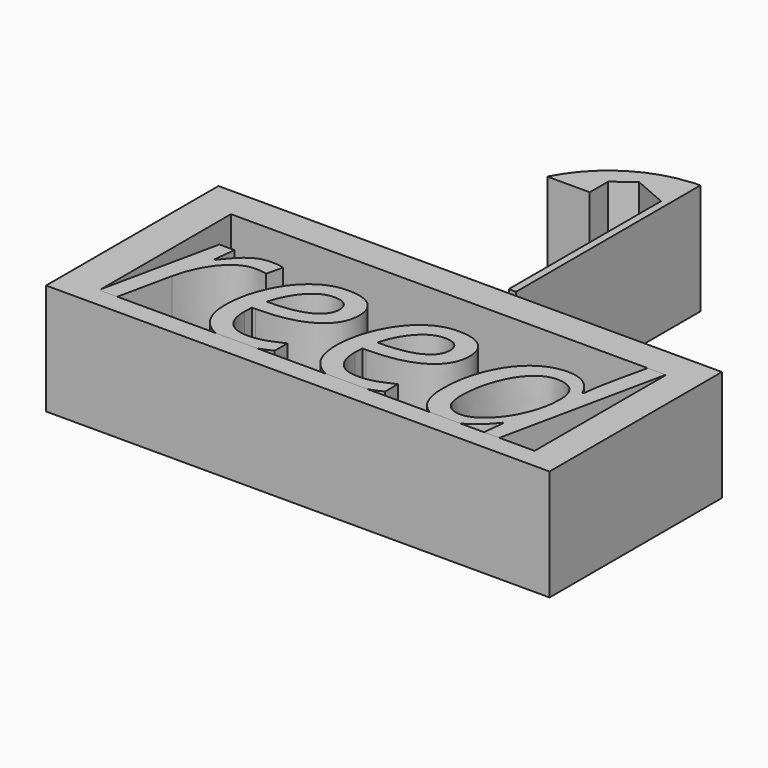
from build123d import *

# Parameters (mm, degrees)
F0_TEXT_SIZE = 51.2880169683
F1_DEPTH     = 25.4
F2_W         = 93.4035778046
F2_H         = 4.566386342
F2_W_2       = 6.2408708036
F2_W_3       = 99.6444486082
F2_H_2       = 7.1163624525
F2_W_4       = 1.6946494579
F2_W_5       = 7.0808120072
F3_DEPTH     = 25.4
F5_DEPTH     = 25.4


# Not quite as in the source:
# - Text() gives the source's letters only with a copy of the font that has no kerning and outlines rounded to 1/6400 em; it was checked with that copy


with BuildPart() as f1:
    # F0 (on Top) → F1 (new body)
    with BuildSketch(Plane.XY):
        with Locations((-53.9388656616, -75.9293287992)):
            Text('reed', F0_TEXT_SIZE, font='Open Sans', font_style=FontStyle.ITALIC, text_align=(TextAlign.LEFT, TextAlign.BOTTOM))
    extrude(amount=F1_DEPTH)


with BuildPart() as f3:
    # F2 (on Top) → F3 (new body)
    with BuildSketch(Plane.XY):
        with Locations((-5.6042224169, -77.9533907771)):
            Rectangle(F2_W, F2_H)
        Polygon((-52.3060113192, -80.2365839481), (-52.3060113192, -75.6701976061), (-52.3060113192, -38.0187183619), (-54.0006607771, -38.0187183619), (-54.0006607771, -80.2365839481), align=None)
        with Locations((44.2180018872, -77.9533907771)):
            Rectangle(F2_W_2, F2_H)
        with Locations((-2.4837870151, -34.4605371356)):
            Rectangle(F2_W_3, F2_H_2)
        with Locations((-53.1533360481, -34.4605371356)):
            Rectangle(F2_W_4, F2_H_2)
        Polygon((47.338437289, -38.0187183619), (47.338437289, -75.6701976061), (47.338437289, -80.2365839481), (54.4192492962, -80.2365839481), (54.4192492962, -38.0187183619), align=None)
        Polygon((-60.8616806567, -80.2365839481), (-54.0006607771, -80.2365839481), (-54.0006607771, -38.0187183619), (-54.0006607771, -30.9023559093), (-60.8616806567, -30.9023559093), align=None)
        with Locations((50.8788432926, -34.4605371356)):
            Rectangle(F2_W_5, F2_H_2)
    extrude(amount=F3_DEPTH)


with BuildPart() as f5:
    # F4 (on Top) → F5 (new body)
    with BuildSketch(Plane.XY):
        with BuildLine():
            Line((4.6046972275, -29.6465158463), (6.2791258097, -29.6465158463))
            Line((6.2791258097, -29.6465158463), (6.2791258097, 23.0982899666))
            ThreePointArc((6.2791258097, 23.0982899666), (5.441488901, 23.0849841514), (4.6046972275, 23.0450801326))
            Line((4.6046972275, 23.0450801326), (4.6046972275, 13.9426963335))
            Line((4.6046972275, 13.9426963335), (4.6046972275, -29.6465158463))
        make_face()
        with BuildLine():
            ThreePointArc((4.6046972275, 23.0450801326), (5.441488901, 23.0849841514), (6.2791258097, 23.0982899666))
            Line((6.2791258097, 23.0982899666), (4.6046972275, 23.0982899666))
            Line((4.6046972275, 23.0982899666), (4.6046972275, 23.0450801326))
        make_face()
        with BuildLine():
            Line((-3.0875055252, 17.2848684449), (4.6046972275, 13.9426963335))
            Line((4.6046972275, 13.9426963335), (4.6046972275, 23.0450801326))
            ThreePointArc((4.6046972275, 23.0450801326), (4.5661746808, 23.0426010171), (4.5276558042, 23.0400655174))
            Line((4.5276558042, 23.0400655174), (-3.0875055252, 17.2848684449))
        make_face()
        with BuildLine():
            Line((4.6046972275, 23.0450801326), (4.6046972275, 23.0982899666))
            Line((4.6046972275, 23.0982899666), (4.5276558042, 23.0400655174))
            ThreePointArc((4.5276558042, 23.0400655174), (4.5661746808, 23.0426010171), (4.6046972275, 23.0450801326))
        make_face()
        Polygon((-7.5098006262, 13.9426963335), (-3.0875055252, 17.2848684449), (-7.5098006262, 19.2063039336), align=None)
        with BuildLine():
            Line((-7.5098006262, 19.2063039336), (-3.0875055252, 17.2848684449))
            Line((-3.0875055252, 17.2848684449), (4.5276558042, 23.0400655174))
            ThreePointArc((4.5276558042, 23.0400655174), (-1.7240243426, 21.8546200704), (-7.5098006262, 19.2063039336))
        make_face()
        with BuildLine():
            Line((-7.5098006262, 13.9426963335), (-7.5098006262, 19.2063039336))
            ThreePointArc((-7.5098006262, 19.2063039336), (-13.0979267677, 14.6153663279), (-17.2288431544, 8.6790887335))
            Line((-17.2288431544, 8.6790887335), (-7.5098006262, 8.6790887335))
            Line((-7.5098006262, 8.6790887335), (-7.5098006262, 13.9426963335))
        make_face()
    extrude(amount=F5_DEPTH)


solid = Compound([f1.part, f3.part, f5.part])
